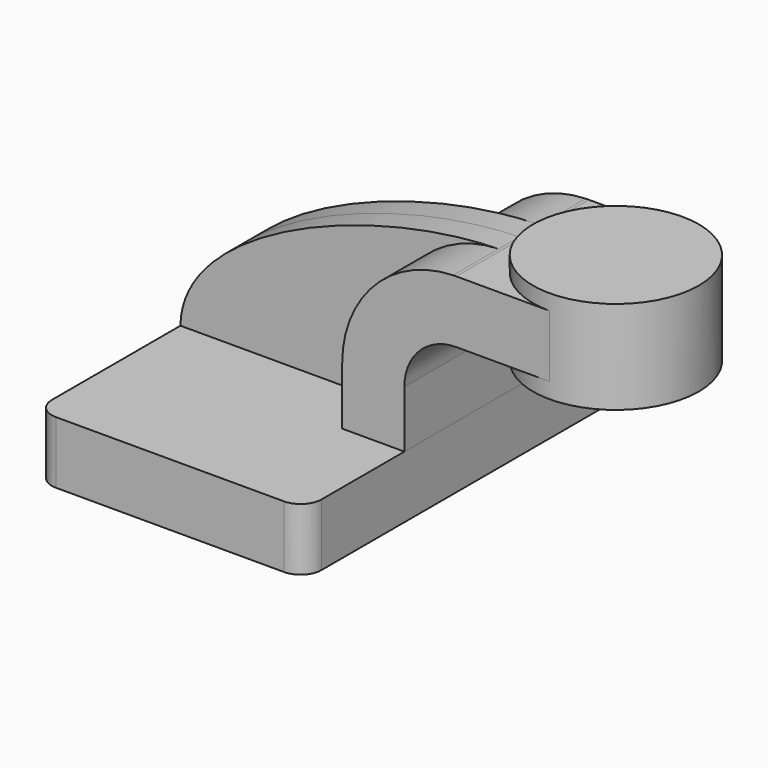
from build123d import *

# Parameters (mm, degrees)
F1_DEPTH = 63.5
F0_W     = 25.4
F0_H     = 19.05
F2_DEPTH = 25.4
F3_DEPTH = 7.9375
F5_R     = 6.35


with BuildPart() as f1:
    # F0 (on Front) → F1 (new body, symmetric)
    with BuildSketch(Plane.XZ):
        Polygon((-41.275, -9.525), (41.275, -9.525), (41.275, 9.525), (22.225, 9.525), (-41.275, 9.525), align=None)
    extrude(amount=F1_DEPTH, both=True)

    # F0 (on Front) → F3 (join, symmetric)
    with BuildSketch(Plane.XZ):
        with BuildLine():
            add(Edge.make_bspline(
                [(-41.275, 9.525), (-40.9770567973, 38.2124460487), (16.4634570461, 61.2015549145), (56.2082941288, 61.9125017725)],
                knots=[0, 0, 0, 0, 110.6276774511, 110.6276774511, 110.6276774511, 110.6276774511], degree=3))
            Line((-41.275, 9.525), (22.225, 9.525))
            Line((22.225, 9.525), (22.225, 27.0002))
            ThreePointArc((22.225, 27.0002), (32.1235669486, 51.360685909), (56.2082941288, 61.9125017725))
        make_face()
    extrude(amount=F3_DEPTH, both=True)

    # F5
    f5_edges = [f1.edges().sort_by_distance(p)[0] for p in [
        (41.275, -63.5, 0),
        (-41.275, -63.5, 0),
        (41.275, 63.5, 0),
        (-41.275, 63.5, 0),
    ]]
    fillet(f5_edges, radius=F5_R)


with BuildPart() as f2:
    # F0 (on Front) → F2 (new body, symmetric)
    with BuildSketch(Plane.XZ):
        with BuildLine():
            Line((22.225, 9.525), (41.275, 9.525))
            Line((41.275, 9.525), (41.275, 27.0002))
            ThreePointArc((41.275, 27.0002), (45.9246798487, 38.2255201513), (57.15, 42.8752))
            Line((57.15, 42.8752), (60.325, 42.8752))
            Line((60.325, 42.8752), (60.325, 61.9252))
            Line((60.325, 61.9252), (57.15, 61.9252))
            add(Edge.make_bspline(
                [(56.2082941288, 61.9125017725), (56.5233202368, 61.9181368898), (56.8372346161, 61.9223723844), (57.15, 61.9252)],
                knots=[110.6276774511, 110.6276774511, 110.6276774511, 110.6276774511, 111.5045361635, 111.5045361635, 111.5045361635, 111.5045361635], degree=3))
            ThreePointArc((56.2082941288, 61.9125017725), (32.1235669486, 51.360685909), (22.225, 27.0002))
            Line((22.225, 27.0002), (22.225, 9.525))
        make_face()
        with Locations((73.025, 52.4002)):
            Rectangle(F0_W, F0_H)
    extrude(amount=F2_DEPTH, both=True)

    # F0 (on Front) → F4 (revolve)
    with BuildSketch(Plane.XZ):
        Polygon((85.725, 61.9252), (85.725, 42.8752), (85.725, 38.1), (111.125, 38.1), (111.125, 66.675), (85.725, 66.675), align=None)
    revolve(axis=Axis((85.725, 0, 52.3875), (0, 0, 1)))


solid = Compound([f1.part, f2.part])
